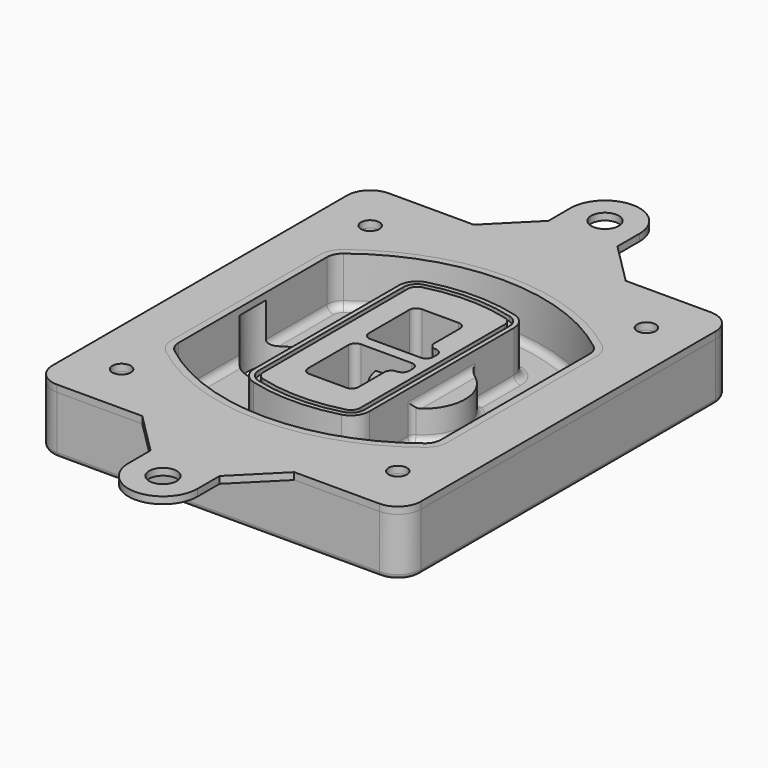
from build123d import *

# Parameters (mm, degrees)
F0_R      = 4
F1_DEPTH  = 25
F2_DEPTH  = 3
F3_DEPTH  = 18
F5_DEPTH  = 21
F6_DEPTH  = 2
F8_DEPTH  = 20
F9_DEPTH  = 16
F10_DEPTH = 25
F7_R      = 6
F7_R_2    = 4
F11_DEPTH = 6
F13_DEPTH = 9
F14_R     = 3
F15_R     = 2
F16_R     = 4
F16_R_2   = 6
F17_DEPTH = 3


# Not quite as in the source:
# - a feature names something its author has since deleted; it is built from what else it names


with BuildPart() as f1:
    # F0 (on Top) → F1 (new body)
    with BuildSketch(Plane.XY):
        with BuildLine():
            ThreePointArc((-80, -80), (-77.0710678119, -87.0710678119), (-70, -90))
            Line((-70, -90), (70, -90))
            ThreePointArc((70, -90), (77.0710678119, -87.0710678119), (80, -80))
            Line((80, -80), (80, 80))
            ThreePointArc((80, 80), (77.0710678119, 87.0710678119), (70, 90))
            Line((70, 90), (-70, 90))
            ThreePointArc((-70, 90), (-77.0710678119, 87.0710678119), (-80, 80))
            Line((-80, 80), (-80, -80))
        make_face()
        with Locations((-60, -67.5)):
            Circle(F0_R, mode=Mode.SUBTRACT)
        with Locations((60, -67.5)):
            Circle(F0_R, mode=Mode.SUBTRACT)
        with Locations((-60, 67.5)):
            Circle(F0_R, mode=Mode.SUBTRACT)
        with BuildLine():
            ThreePointArc((-64, 40.2934422872), (-62.5820384798, 46.4328484224), (-58.6153846154, 51.3286200352))
            ThreePointArc((-58.6153846154, 51.3286200352), (0, 71.5), (58.6153846154, 51.3286200352))
            ThreePointArc((58.6153846154, 51.3286200352), (62.5820384798, 46.4328484224), (64, 40.2934422872))
            Line((64, 40.2934422872), (64, -40.2934422872))
            ThreePointArc((64, -40.2934422872), (62.5820384798, -46.4328484224), (58.6153846154, -51.3286200352))
            ThreePointArc((58.6153846154, -51.3286200352), (0, -71.5), (-58.6153846154, -51.3286200352))
            ThreePointArc((-58.6153846154, -51.3286200352), (-62.5820384798, -46.4328484224), (-64, -40.2934422872))
            Line((-64, -40.2934422872), (-64, 40.2934422872))
        make_face(mode=Mode.SUBTRACT)
        with Locations((60, 67.5)):
            Circle(F0_R, mode=Mode.SUBTRACT)
        with BuildLine():
            ThreePointArc((58.6153846154, 51.3286200352), (0, 71.5), (-58.6153846154, 51.3286200352))
            ThreePointArc((-58.6153846154, 51.3286200352), (-62.5820384798, 46.4328484224), (-64, 40.2934422872))
            Line((-64, 40.2934422872), (-64, -40.2934422872))
            ThreePointArc((-64, -40.2934422872), (-62.5820384798, -46.4328484224), (-58.6153846154, -51.3286200352))
            ThreePointArc((-58.6153846154, -51.3286200352), (0, -71.5), (58.6153846154, -51.3286200352))
            ThreePointArc((58.6153846154, -51.3286200352), (62.5820384798, -46.4328484224), (64, -40.2934422872))
            Line((64, -40.2934422872), (64, 40.2934422872))
            ThreePointArc((64, 40.2934422872), (62.5820384798, 46.4328484224), (58.6153846154, 51.3286200352))
        make_face()
        with BuildLine():
            Line((-60, -40.2934422872), (-60, 40.2934422872))
            ThreePointArc((-60, 40.2934422872), (-58.9871703427, 44.6787323838), (-56.1538461538, 48.1757121072))
            ThreePointArc((-56.1538461538, 48.1757121072), (0, 67.5), (56.1538461538, 48.1757121072))
            ThreePointArc((56.1538461538, 48.1757121072), (58.9871703427, 44.6787323838), (60, 40.2934422872))
            Line((60, 40.2934422872), (60, -40.2934422872))
            ThreePointArc((60, -40.2934422872), (58.9871703427, -44.6787323838), (56.1538461538, -48.1757121072))
            ThreePointArc((56.1538461538, -48.1757121072), (0, -67.5), (-56.1538461538, -48.1757121072))
            ThreePointArc((-56.1538461538, -48.1757121072), (-58.9871703427, -44.6787323838), (-60, -40.2934422872))
        make_face(mode=Mode.SUBTRACT)
        with BuildLine():
            ThreePointArc((-56.1538461538, 48.1757121072), (-58.9871703427, 44.6787323838), (-60, 40.2934422872))
            Line((-60, 40.2934422872), (-60, -40.2934422872))
            ThreePointArc((-60, -40.2934422872), (-58.9871703427, -44.6787323838), (-56.1538461538, -48.1757121072))
            ThreePointArc((-56.1538461538, -48.1757121072), (0, -67.5), (56.1538461538, -48.1757121072))
            ThreePointArc((56.1538461538, -48.1757121072), (58.9871703427, -44.6787323838), (60, -40.2934422872))
            Line((60, -40.2934422872), (60, 40.2934422872))
            ThreePointArc((60, 40.2934422872), (58.9871703427, 44.6787323838), (56.1538461538, 48.1757121072))
            ThreePointArc((56.1538461538, 48.1757121072), (0, 67.5), (-56.1538461538, 48.1757121072))
        make_face()
        with BuildLine():
            ThreePointArc((54.3076923077, 45.8110311612), (56.2910192399, 43.3631453548), (57, 40.2934422872))
            Line((57, 40.2934422872), (57, -40.2934422872))
            ThreePointArc((57, -40.2934422872), (56.2910192399, -43.3631453548), (54.3076923077, -45.8110311612))
            ThreePointArc((54.3076923077, -45.8110311612), (0, -64.5), (-54.3076923077, -45.8110311612))
            ThreePointArc((-54.3076923077, -45.8110311612), (-56.2910192399, -43.3631453548), (-57, -40.2934422872))
            Line((-57, -40.2934422872), (-57, 40.2934422872))
            ThreePointArc((-57, 40.2934422872), (-56.2910192399, 43.3631453548), (-54.3076923077, 45.8110311612))
            ThreePointArc((-54.3076923077, 45.8110311612), (0, 64.5), (54.3076923077, 45.8110311612))
        make_face(mode=Mode.SUBTRACT)
        with BuildLine():
            Line((57, -40.2934422872), (57, 40.2934422872))
            ThreePointArc((57, 40.2934422872), (56.2910192399, 43.3631453548), (54.3076923077, 45.8110311612))
            ThreePointArc((54.3076923077, 45.8110311612), (0, 64.5), (-54.3076923077, 45.8110311612))
            ThreePointArc((-54.3076923077, 45.8110311612), (-56.2910192399, 43.3631453548), (-57, 40.2934422872))
            Line((-57, 40.2934422872), (-57, -40.2934422872))
            ThreePointArc((-57, -40.2934422872), (-56.2910192399, -43.3631453548), (-54.3076923077, -45.8110311612))
            ThreePointArc((-54.3076923077, -45.8110311612), (0, -64.5), (54.3076923077, -45.8110311612))
            ThreePointArc((54.3076923077, -45.8110311612), (56.2910192399, -43.3631453548), (57, -40.2934422872))
        make_face()
    extrude(amount=-F1_DEPTH)

    # F0 (on Top) → F2 (join)
    with BuildSketch(Plane.XY):
        with BuildLine():
            ThreePointArc((-56.1538461538, 48.1757121072), (-58.9871703427, 44.6787323838), (-60, 40.2934422872))
            Line((-60, 40.2934422872), (-60, -40.2934422872))
            ThreePointArc((-60, -40.2934422872), (-58.9871703427, -44.6787323838), (-56.1538461538, -48.1757121072))
            ThreePointArc((-56.1538461538, -48.1757121072), (0, -67.5), (56.1538461538, -48.1757121072))
            ThreePointArc((56.1538461538, -48.1757121072), (58.9871703427, -44.6787323838), (60, -40.2934422872))
            Line((60, -40.2934422872), (60, 40.2934422872))
            ThreePointArc((60, 40.2934422872), (58.9871703427, 44.6787323838), (56.1538461538, 48.1757121072))
            ThreePointArc((56.1538461538, 48.1757121072), (0, 67.5), (-56.1538461538, 48.1757121072))
        make_face()
        with BuildLine():
            ThreePointArc((54.3076923077, 45.8110311612), (56.2910192399, 43.3631453548), (57, 40.2934422872))
            Line((57, 40.2934422872), (57, -40.2934422872))
            ThreePointArc((57, -40.2934422872), (56.2910192399, -43.3631453548), (54.3076923077, -45.8110311612))
            ThreePointArc((54.3076923077, -45.8110311612), (0, -64.5), (-54.3076923077, -45.8110311612))
            ThreePointArc((-54.3076923077, -45.8110311612), (-56.2910192399, -43.3631453548), (-57, -40.2934422872))
            Line((-57, -40.2934422872), (-57, 40.2934422872))
            ThreePointArc((-57, 40.2934422872), (-56.2910192399, 43.3631453548), (-54.3076923077, 45.8110311612))
            ThreePointArc((-54.3076923077, 45.8110311612), (0, 64.5), (54.3076923077, 45.8110311612))
        make_face(mode=Mode.SUBTRACT)
    extrude(amount=F2_DEPTH)

    # F0 (on Top) → F3 (cut)
    with BuildSketch(Plane.XY):
        with BuildLine():
            Line((57, -40.2934422872), (57, 40.2934422872))
            ThreePointArc((57, 40.2934422872), (56.2910192399, 43.3631453548), (54.3076923077, 45.8110311612))
            ThreePointArc((54.3076923077, 45.8110311612), (0, 64.5), (-54.3076923077, 45.8110311612))
            ThreePointArc((-54.3076923077, 45.8110311612), (-56.2910192399, 43.3631453548), (-57, 40.2934422872))
            Line((-57, 40.2934422872), (-57, -40.2934422872))
            ThreePointArc((-57, -40.2934422872), (-56.2910192399, -43.3631453548), (-54.3076923077, -45.8110311612))
            ThreePointArc((-54.3076923077, -45.8110311612), (0, -64.5), (54.3076923077, -45.8110311612))
            ThreePointArc((54.3076923077, -45.8110311612), (56.2910192399, -43.3631453548), (57, -40.2934422872))
        make_face()
    extrude(amount=-F3_DEPTH, mode=Mode.SUBTRACT)

    # F4 (on face) → F5 (join, through all)
    with BuildSketch(Plane.XY.offset(3)):
        with BuildLine():
            ThreePointArc((-25, -39.2465276821), (-23.3511545998, -44.1109737193), (-19.0842911877, -46.9702398883))
            ThreePointArc((-19.0842911877, -46.9702398883), (0, -49.5), (19.0842911877, -46.9702398883))
            ThreePointArc((19.0842911877, -46.9702398883), (23.3511545998, -44.1109737193), (25, -39.2465276821))
            Line((25, -39.2465276821), (25, 39.2465276821))
            ThreePointArc((25, 39.2465276821), (23.3511545998, 44.1109737193), (19.0842911877, 46.9702398883))
            ThreePointArc((19.0842911877, 46.9702398883), (0, 49.5), (-19.0842911877, 46.9702398883))
            ThreePointArc((-19.0842911877, 46.9702398883), (-23.3511545998, 44.1109737193), (-25, 39.2465276821))
            Line((-25, 39.2465276821), (-25, -39.2465276821))
        make_face()
        with BuildLine():
            ThreePointArc((18.5632183908, 45.0393118368), (21.7633659499, 42.89486221), (23, 39.2465276821))
            Line((23, 39.2465276821), (23, -39.2465276821))
            ThreePointArc((23, -39.2465276821), (21.7633659499, -42.89486221), (18.5632183908, -45.0393118368))
            ThreePointArc((18.5632183908, -45.0393118368), (0, -47.5), (-18.5632183908, -45.0393118368))
            ThreePointArc((-18.5632183908, -45.0393118368), (-21.7633659499, -42.89486221), (-23, -39.2465276821))
            Line((-23, -39.2465276821), (-23, 39.2465276821))
            ThreePointArc((-23, 39.2465276821), (-21.7633659499, 42.89486221), (-18.5632183908, 45.0393118368))
            ThreePointArc((-18.5632183908, 45.0393118368), (0, 47.5), (18.5632183908, 45.0393118368))
        make_face(mode=Mode.SUBTRACT)
        with BuildLine():
            Line((23, -39.2465276821), (23, 39.2465276821))
            ThreePointArc((23, 39.2465276821), (21.7633659499, 42.89486221), (18.5632183908, 45.0393118368))
            ThreePointArc((18.5632183908, 45.0393118368), (0, 47.5), (-18.5632183908, 45.0393118368))
            ThreePointArc((-18.5632183908, 45.0393118368), (-21.7633659499, 42.89486221), (-23, 39.2465276821))
            Line((-23, 39.2465276821), (-23, -39.2465276821))
            ThreePointArc((-23, -39.2465276821), (-21.7633659499, -42.89486221), (-18.5632183908, -45.0393118368))
            ThreePointArc((-18.5632183908, -45.0393118368), (0, -47.5), (18.5632183908, -45.0393118368))
            ThreePointArc((18.5632183908, -45.0393118368), (21.7633659499, -42.89486221), (23, -39.2465276821))
        make_face()
        with BuildLine():
            ThreePointArc((18.0421455939, 43.1083837852), (20.1755772999, 41.6787507007), (21, 39.2465276821))
            Line((21, 39.2465276821), (21, -39.2465276821))
            ThreePointArc((21, -39.2465276821), (20.1755772999, -41.6787507007), (18.0421455939, -43.1083837852))
            ThreePointArc((18.0421455939, -43.1083837852), (0, -45.5), (-18.0421455939, -43.1083837852))
            ThreePointArc((-18.0421455939, -43.1083837852), (-20.1755772999, -41.6787507007), (-21, -39.2465276821))
            Line((-21, -39.2465276821), (-21, 39.2465276821))
            ThreePointArc((-21, 39.2465276821), (-20.1755772999, 41.6787507007), (-18.0421455939, 43.1083837852))
            ThreePointArc((-18.0421455939, 43.1083837852), (0, 45.5), (18.0421455939, 43.1083837852))
        make_face(mode=Mode.SUBTRACT)
        with BuildLine():
            Line((21, -39.2465276821), (21, 39.2465276821))
            ThreePointArc((21, 39.2465276821), (20.1755772999, 41.6787507007), (18.0421455939, 43.1083837852))
            ThreePointArc((18.0421455939, 43.1083837852), (0, 45.5), (-18.0421455939, 43.1083837852))
            ThreePointArc((-18.0421455939, 43.1083837852), (-20.1755772999, 41.6787507007), (-21, 39.2465276821))
            Line((-21, 39.2465276821), (-21, -39.2465276821))
            ThreePointArc((-21, -39.2465276821), (-20.1755772999, -41.6787507007), (-18.0421455939, -43.1083837852))
            ThreePointArc((-18.0421455939, -43.1083837852), (0, -45.5), (18.0421455939, -43.1083837852))
            ThreePointArc((18.0421455939, -43.1083837852), (20.1755772999, -41.6787507007), (21, -39.2465276821))
        make_face()
        with BuildLine():
            Line((-8, -2.5), (14, -2.5))
            ThreePointArc((14, -2.5), (16.1213203436, -3.3786796564), (17, -5.5))
            Line((17, -5.5), (17, -7.5))
            ThreePointArc((17, -7.5), (16.1213203436, -9.6213203436), (14, -10.5))
            ThreePointArc((14, -10.5), (11.8786796564, -11.3786796564), (11, -13.5))
            Line((11, -13.5), (11, -27.5))
            ThreePointArc((11, -27.5), (10.1213203436, -29.6213203436), (8, -30.5))
            Line((8, -30.5), (-8, -30.5))
            ThreePointArc((-8, -30.5), (-10.1213203436, -29.6213203436), (-11, -27.5))
            Line((-11, -27.5), (-11, -5.5))
            ThreePointArc((-11, -5.5), (-10.1213203436, -3.3786796564), (-8, -2.5))
        make_face(mode=Mode.SUBTRACT)
        with BuildLine():
            ThreePointArc((-8, 2.5), (-10.1213203436, 3.3786796564), (-11, 5.5))
            Line((-11, 5.5), (-11, 27.5))
            ThreePointArc((-11, 27.5), (-10.1213203436, 29.6213203436), (-8, 30.5))
            Line((-8, 30.5), (8, 30.5))
            ThreePointArc((8, 30.5), (10.1213203436, 29.6213203436), (11, 27.5))
            Line((11, 27.5), (11, 13.5))
            ThreePointArc((11, 13.5), (11.8786796564, 11.3786796564), (14, 10.5))
            ThreePointArc((14, 10.5), (16.1213203436, 9.6213203436), (17, 7.5))
            Line((17, 7.5), (17, 5.5))
            ThreePointArc((17, 5.5), (16.1213203436, 3.3786796564), (14, 2.5))
            Line((14, 2.5), (-8, 2.5))
        make_face(mode=Mode.SUBTRACT)
    extrude(amount=-F5_DEPTH)

    # F4 (on face) → F6 (cut)
    with BuildSketch(Plane.XY.offset(3)):
        with BuildLine():
            Line((23, -39.2465276821), (23, 39.2465276821))
            ThreePointArc((23, 39.2465276821), (21.7633659499, 42.89486221), (18.5632183908, 45.0393118368))
            ThreePointArc((18.5632183908, 45.0393118368), (0, 47.5), (-18.5632183908, 45.0393118368))
            ThreePointArc((-18.5632183908, 45.0393118368), (-21.7633659499, 42.89486221), (-23, 39.2465276821))
            Line((-23, 39.2465276821), (-23, -39.2465276821))
            ThreePointArc((-23, -39.2465276821), (-21.7633659499, -42.89486221), (-18.5632183908, -45.0393118368))
            ThreePointArc((-18.5632183908, -45.0393118368), (0, -47.5), (18.5632183908, -45.0393118368))
            ThreePointArc((18.5632183908, -45.0393118368), (21.7633659499, -42.89486221), (23, -39.2465276821))
        make_face()
        with BuildLine():
            ThreePointArc((18.0421455939, 43.1083837852), (20.1755772999, 41.6787507007), (21, 39.2465276821))
            Line((21, 39.2465276821), (21, -39.2465276821))
            ThreePointArc((21, -39.2465276821), (20.1755772999, -41.6787507007), (18.0421455939, -43.1083837852))
            ThreePointArc((18.0421455939, -43.1083837852), (0, -45.5), (-18.0421455939, -43.1083837852))
            ThreePointArc((-18.0421455939, -43.1083837852), (-20.1755772999, -41.6787507007), (-21, -39.2465276821))
            Line((-21, -39.2465276821), (-21, 39.2465276821))
            ThreePointArc((-21, 39.2465276821), (-20.1755772999, 41.6787507007), (-18.0421455939, 43.1083837852))
            ThreePointArc((-18.0421455939, 43.1083837852), (0, 45.5), (18.0421455939, 43.1083837852))
        make_face(mode=Mode.SUBTRACT)
    extrude(amount=-F6_DEPTH, mode=Mode.SUBTRACT)

    # F7 (on face) → F8 (join)
    with BuildSketch(Plane(origin=(0, 0, -25), x_dir=(1, 0, 0), z_dir=(0, 0, -1))):
        with BuildLine():
            ThreePointArc((3.28842436, 0), (16.7567035675, 13.4682792075), (30.224982775, 0))
            Line((30.224982775, 0), (35.224982775, 0))
            ThreePointArc((35.224982775, 0), (16.7567035675, 18.4682792075), (-1.71157564, 0))
            Line((-1.71157564, 0), (3.28842436, 0))
        make_face()
        with BuildLine():
            Line((3.28842436, 0), (30.224982775, 0))
            ThreePointArc((30.224982775, 0), (16.7567035675, 13.4682792075), (3.28842436, 0))
        make_face()
        with BuildLine():
            ThreePointArc((3.28842436, 0), (16.7567035675, -13.4682792075), (30.224982775, 0))
            Line((30.224982775, 0), (3.28842436, 0))
        make_face()
        with BuildLine():
            Line((35.224982775, 0), (30.224982775, 0))
            ThreePointArc((30.224982775, 0), (16.7567035675, -13.4682792075), (3.28842436, 0))
            Line((3.28842436, 0), (-1.71157564, 0))
            ThreePointArc((-1.71157564, 0), (16.7567035675, -18.4682792075), (35.224982775, 0))
        make_face()
    extrude(amount=-F8_DEPTH)

    # F7 (on face) → F9 (cut)
    with BuildSketch(Plane(origin=(0, 0, -25), x_dir=(1, 0, 0), z_dir=(0, 0, -1))):
        with BuildLine():
            Line((3.28842436, 0), (30.224982775, 0))
            ThreePointArc((30.224982775, 0), (16.7567035675, 13.4682792075), (3.28842436, 0))
        make_face()
        with BuildLine():
            ThreePointArc((3.28842436, 0), (16.7567035675, -13.4682792075), (30.224982775, 0))
            Line((30.224982775, 0), (3.28842436, 0))
        make_face()
    extrude(amount=-F9_DEPTH, mode=Mode.SUBTRACT)

    # F7 (on face) → F10 (cut)
    with BuildSketch(Plane(origin=(0, 0, -25), x_dir=(1, 0, 0), z_dir=(0, 0, -1))):
        with BuildLine():
            Line((-59.0318229325, 0), (-32.0952645175, 0))
            ThreePointArc((-32.0952645175, 0), (-45.563543725, 13.4682792075), (-59.0318229325, 0))
        make_face()
        with BuildLine():
            ThreePointArc((-59.0318229325, 0), (-45.563543725, -13.4682792075), (-32.0952645175, 0))
            Line((-32.0952645175, 0), (-59.0318229325, 0))
        make_face()
    extrude(amount=-F10_DEPTH, mode=Mode.SUBTRACT)

    # F7 (on face) → F11 (cut)
    with BuildSketch(Plane(origin=(0, 0, -25), x_dir=(1, 0, 0), z_dir=(0, 0, -1))):
        with Locations((60, -67.5)):
            Circle(F7_R)
        with Locations((60, -67.5)):
            Circle(F7_R_2, mode=Mode.SUBTRACT)
        with Locations((-60, -67.5)):
            Circle(F7_R)
        with Locations((-60, -67.5)):
            Circle(F7_R_2, mode=Mode.SUBTRACT)
        with Locations((-60, 67.5)):
            Circle(F7_R)
        with Locations((-60, 67.5)):
            Circle(F7_R_2, mode=Mode.SUBTRACT)
        with Locations((60, 67.5)):
            Circle(F7_R)
        with Locations((60, 67.5)):
            Circle(F7_R_2, mode=Mode.SUBTRACT)
    extrude(amount=-F11_DEPTH, mode=Mode.SUBTRACT)

    # F12 (on face) → F13 (cut, through all)
    with BuildSketch(Plane(origin=(0, 0, -9), x_dir=(1, 0, 0), z_dir=(0, 0, -1))):
        with BuildLine():
            Line((11, 13.5), (11, 17.5481537753))
            ThreePointArc((11, 17.5481537753), (2.5696536419, 11.8239143813), (-1.5415842455, 2.5))
            Line((-1.5415842455, 2.5), (3.5224848595, 2.5))
            ThreePointArc((3.5224848595, 2.5), (6.1857188154, 8.3455872281), (11.2536447004, 12.2927168648))
            ThreePointArc((11.2536447004, 12.2927168648), (11.0640958889, 12.8831798879), (11, 13.5))
        make_face()
        with BuildLine():
            ThreePointArc((11.2536447004, -12.2927168648), (6.1857188154, -8.3455872281), (3.5224848595, -2.5))
            Line((3.5224848595, -2.5), (-1.5415842455, -2.5))
            ThreePointArc((-1.5415842455, -2.5), (2.5696536419, -11.8239143813), (11, -17.5481537753))
            Line((11, -17.5481537753), (11, -13.5))
            ThreePointArc((11, -13.5), (11.0640958889, -12.8831798879), (11.2536447004, -12.2927168648))
        make_face()
        with BuildLine():
            ThreePointArc((11.2536447004, 12.2927168648), (6.1857188154, 8.3455872281), (3.5224848595, 2.5))
            Line((3.5224848595, 2.5), (14, 2.5))
            ThreePointArc((14, 2.5), (16.1213203436, 3.3786796564), (17, 5.5))
            Line((17, 5.5), (17, 7.5))
            ThreePointArc((17, 7.5), (16.1213203436, 9.6213203436), (14, 10.5))
            ThreePointArc((14, 10.5), (12.3601599782, 10.9878446101), (11.2536447004, 12.2927168648))
        make_face()
        with BuildLine():
            Line((14, -2.5), (3.5224848595, -2.5))
            ThreePointArc((3.5224848595, -2.5), (6.1857188154, -8.3455872281), (11.2536447004, -12.2927168648))
            ThreePointArc((11.2536447004, -12.2927168648), (12.3601599782, -10.9878446101), (14, -10.5))
            ThreePointArc((14, -10.5), (16.1213203436, -9.6213203436), (17, -7.5))
            Line((17, -7.5), (17, -5.5))
            ThreePointArc((17, -5.5), (16.1213203436, -3.3786796564), (14, -2.5))
        make_face()
    extrude(amount=F13_DEPTH, mode=Mode.SUBTRACT)

    # F14
    f14_edges = [f1.edges().sort_by_distance(p)[0] for p in [
        (-57, -23.703476, -18),
        (-57, 23.703476, -18),
        (25, 0, -5),
        (25, 16.526506, -11.5),
        (25, -16.526506, -11.5),
        (25, -27.886517, -18),
        (35.224983, 0, -18),
    ]]
    fillet(f14_edges, radius=F14_R)

    # F15
    f15_edges = [f1.edges().sort_by_distance(p)[0] for p in [
        (0, -90, -25),
    ]]
    fillet(f15_edges, radius=F15_R)


with BuildPart() as f17:
    # F16 (on face) → F17 (new body)
    with BuildSketch(Plane.XY):
        with BuildLine():
            Line((33, 90), (-33, 90))
            Line((-33, 90), (-70, 90))
            ThreePointArc((-70, 90), (-77.0710678119, 87.0710678119), (-80, 80))
            Line((-80, 80), (-80, -80))
            ThreePointArc((-80, -80), (-77.0710678119, -87.0710678119), (-70, -90))
            Line((-70, -90), (-33, -90))
            Line((-33, -90), (33, -90))
            Line((33, -90), (70, -90))
            ThreePointArc((70, -90), (77.0710678119, -87.0710678119), (80, -80))
            Line((80, -80), (80, 80))
            ThreePointArc((80, 80), (77.0710678119, 87.0710678119), (70, 90))
            Line((70, 90), (33, 90))
        make_face()
        with Locations((-60, -67.5)):
            Circle(F16_R, mode=Mode.SUBTRACT)
        with Locations((60, -67.5)):
            Circle(F16_R, mode=Mode.SUBTRACT)
        with Locations((-60, 67.5)):
            Circle(F16_R, mode=Mode.SUBTRACT)
        with BuildLine():
            ThreePointArc((-60, 40.2934422872), (-58.9871703427, 44.6787323838), (-56.1538461538, 48.1757121072))
            ThreePointArc((-56.1538461538, 48.1757121072), (0, 67.5), (56.1538461538, 48.1757121072))
            ThreePointArc((56.1538461538, 48.1757121072), (58.9871703427, 44.6787323838), (60, 40.2934422872))
            Line((60, 40.2934422872), (60, -40.2934422872))
            ThreePointArc((60, -40.2934422872), (58.9871703427, -44.6787323838), (56.1538461538, -48.1757121072))
            ThreePointArc((56.1538461538, -48.1757121072), (0, -67.5), (-56.1538461538, -48.1757121072))
            ThreePointArc((-56.1538461538, -48.1757121072), (-58.9871703427, -44.6787323838), (-60, -40.2934422872))
            Line((-60, -40.2934422872), (-60, 40.2934422872))
        make_face(mode=Mode.SUBTRACT)
        with Locations((60, 67.5)):
            Circle(F16_R, mode=Mode.SUBTRACT)
        with BuildLine():
            Line((33, -90), (-33, -90))
            Line((-33, -90), (-15, -108))
            Line((-15, -108), (-15, -120))
            ThreePointArc((-15, -120), (0, -135), (15, -120))
            Line((15, -120), (15, -108))
            Line((15, -108), (33, -90))
        make_face()
        with Locations((0, -120)):
            Circle(F16_R_2, mode=Mode.SUBTRACT)
        with BuildLine():
            Line((-15, 120), (-15, 108))
            Line((-15, 108), (-33, 90))
            Line((-33, 90), (33, 90))
            Line((33, 90), (15, 108))
            Line((15, 108), (15, 120))
            ThreePointArc((15, 120), (0, 135), (-15, 120))
        make_face()
        with Locations((0, 120)):
            Circle(F16_R_2, mode=Mode.SUBTRACT)
    extrude(amount=F17_DEPTH)


solid = Compound([f1.part, f17.part])
